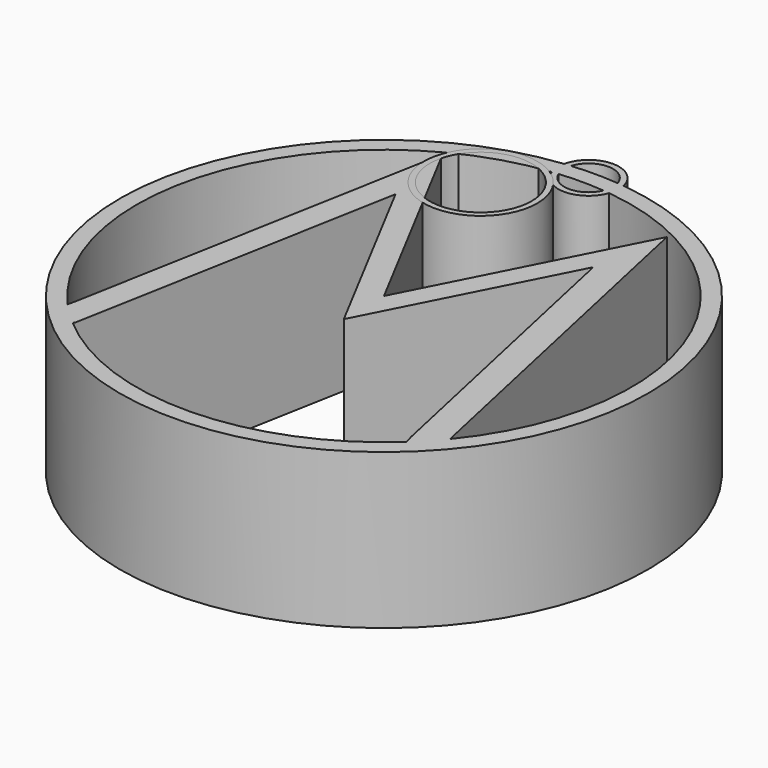
from build123d import *

# Parameters (mm, degrees)
F0_R      = 42.5901202059
F0_R_2    = 39.8982916651
F1_DEPTH  = 25
F3_DEPTH  = 25
F5_DEPTH  = 25
F7_DEPTH  = 25
F8_R      = 4.9005997311
F8_R_2    = 3.9339377278
F9_DEPTH  = 25
F10_R     = 9.1556057754
F10_R_2   = 8.2241228005
F12_DEPTH = 25


# Not quite as in the source:
# - the program builds the solid bodies; features that only make, move or delete a surface that nothing else refers to are left out


with BuildPart() as f1:
    # F0 (on Top) → F1 (new body)
    with BuildSketch(Plane.XY):
        Circle(F0_R)
        Circle(F0_R_2, mode=Mode.SUBTRACT)
    extrude(amount=F1_DEPTH)

    # F2 (on Top) → F3 (join)
    with BuildSketch(Plane.XY):
        Polygon((-18.3799806982, 34.8173640668), (-29.4378567487, -25.5526583642), (-25.8515197784, -30.0355795771), (-16.209538835, 22.6044213756), (0, -8.1014549928), (15.6823994675, 22.6044213756), (26.7224249176, -28.0793387221), (30.932161957, -25.5526583642), (17.7822578698, 34.8173640668), (0, 0), align=None)
    extrude(amount=F3_DEPTH)

    # F4 (on Top) → F5 (join)
    with BuildSketch(Plane.XY):
        Polygon((-25.5759004503, -28.1734243035), (-29.1299819946, -24.0862295032), (-30.0185028464, -28.1734243035), (-26.3755694032, -31.9940634072), align=None)
    extrude(amount=F5_DEPTH)

    # F6 (on Top) → F7 (join)
    with BuildSketch(Plane.XY):
        Polygon((29.9566332251, -24.3527851999), (26.4025498182, -26.485234499), (27.4687726051, -31.0166906565), (30.9340041131, -26.3075307012), align=None)
    extrude(amount=F7_DEPTH)

    # F8 (on Top) → F9 (join)
    with BuildSketch(Plane.XY):
        with Locations((0, 41.2680134177)):
            Circle(F8_R)
        with Locations((0, 41.2680134177)):
            Circle(F8_R_2, mode=Mode.SUBTRACT)
    extrude(amount=F9_DEPTH)


with BuildPart() as f12:
    # F10 (on Top) → F12 (new body)
    with BuildSketch(Plane.XY):
        with Locations((-9.8588764668, 31.8153724074)):
            Circle(F10_R)
        with Locations((-9.8588764668, 31.8153724074)):
            Circle(F10_R_2, mode=Mode.SUBTRACT)
    extrude(amount=F12_DEPTH)


solid = Compound([f1.part, f12.part])
